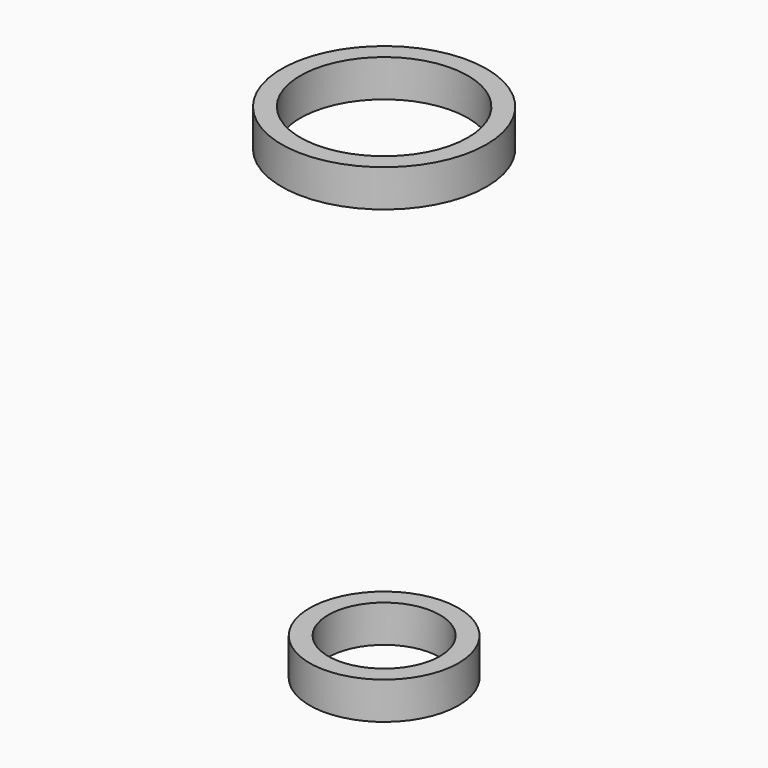
from build123d import *

# Parameters (mm, degrees)
F0_R     = 4
F0_R_2   = 3
F1_DEPTH = 2
F3_R     = 5.5
F3_R_2   = 4.5
F4_DEPTH = 2


with BuildPart() as f1:
    # F0 (on Top) → F1 (new body)
    with BuildSketch(Plane.XY):
        Circle(F0_R)
        Circle(F0_R_2, mode=Mode.SUBTRACT)
    extrude(amount=F1_DEPTH)


with BuildPart() as f4:
    # F3 (on offset) → F4 (new body)
    with BuildSketch(Plane.XY.offset(25)):
        Circle(F3_R)
        Circle(F3_R_2, mode=Mode.SUBTRACT)
    extrude(amount=F4_DEPTH)


solid = Compound([f1.part, f4.part])
